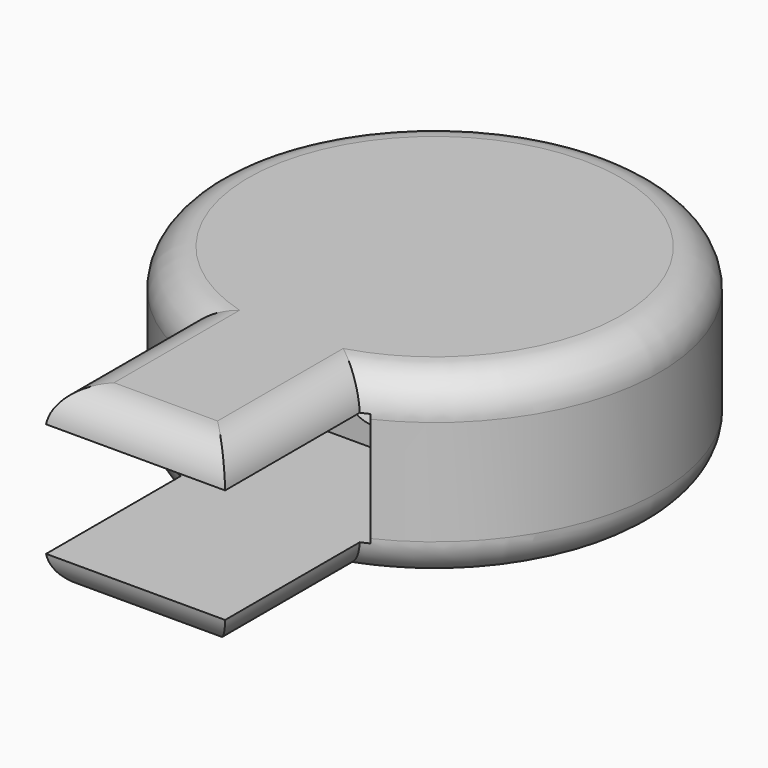
from build123d import *

# Parameters (mm, degrees)
F1_DEPTH = 12.1
F2_R     = 2.53999
F3_W     = 13.0256410256
F3_H     = 7.62
F4_DEPTH = 20
F5_R     = 2.5
F6_DEPTH = 25.4


# Not quite as in the source:
# - a fillet or chamfer is up to 0.001 mm smaller than in the source, because OpenCascade refuses the exact size


with BuildPart() as f1:
    # F0 (on Top) → F1 (new body)
    with BuildSketch(Plane.XY):
        with BuildLine():
            Line((6, -25), (6, -13.7477270849))
            ThreePointArc((6, -13.7477270849), (0, 15), (-6, -13.7477270849))
            Line((-6, -13.7477270849), (-6, -25))
            Line((-6, -25), (0, -25))
            Line((0, -25), (6, -25))
        make_face()
    extrude(amount=F1_DEPTH)

    # F2 (radius 2.54 in the source; OpenCascade refuses exactly that, so slightly less here)
    f2_edges = [f1.edges().sort_by_distance(p)[0] for p in [
        (-6, -19.373864, 12.1),
        (0, -25, 12.1),
        (6, -19.373864, 12.1),
        (0, 15, 12.1),
        (-6, -19.373864, 0),
        (0, -25, 0),
        (6, -19.373864, 0),
        (0, 15, 0),
    ]]
    fillet(f2_edges, radius=F2_R)

    # F3 (on face) → F4 (cut)
    with BuildSketch(Plane.XZ.offset(25)):
        with Locations((0, 6.05)):
            Rectangle(F3_W, F3_H)
    extrude(amount=-F4_DEPTH, mode=Mode.SUBTRACT)

    # F5 (on face) → F6 (cut)
    with BuildSketch(Plane.XZ.offset(5)):
        with Locations((0, 6.05)):
            Circle(F5_R)
    extrude(amount=-F6_DEPTH, mode=Mode.SUBTRACT)


solid = f1.part
